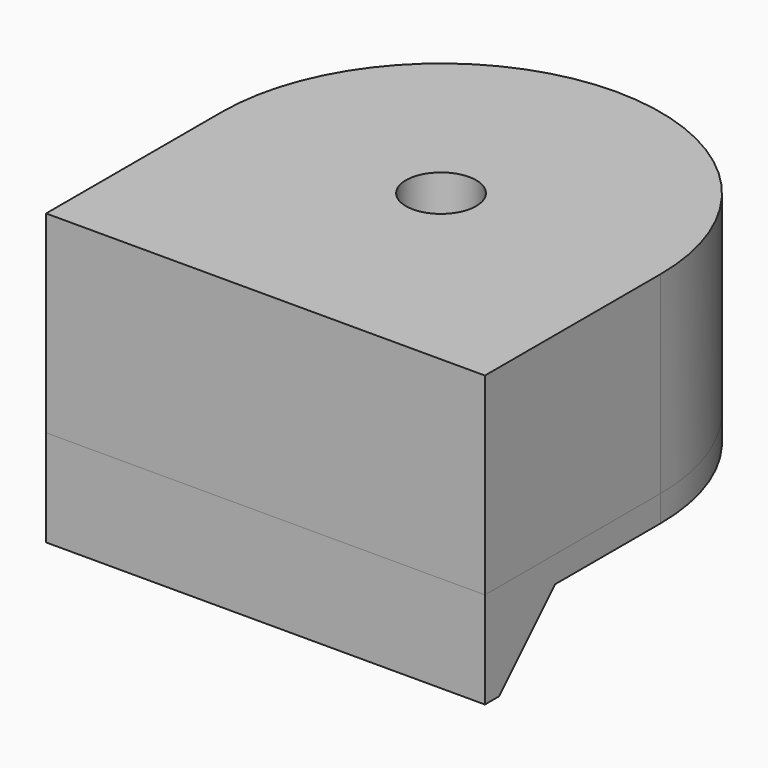
from build123d import *

# Parameters (mm, degrees)
F1_R     = 2
F2_DEPTH = 11
F3_DEPTH = 1.5
F5_DEPTH = 5.5
F6_SIZE  = 3.99999


# Not quite as in the source:
# - a fillet or chamfer is up to 0.001 mm smaller than in the source, because OpenCascade refuses the exact size


with BuildPart() as f2:
    # F1 (on Top) → F2 (new body)
    with BuildSketch(Plane.XY):
        with BuildLine():
            ThreePointArc((-4.8989794856, -11.5), (-10.4280209908, -6.8924870849), (-12.5, 0))
            Line((-12.5, 0), (-12.5, -11.5))
            Line((-12.5, -11.5), (-4.8989794856, -11.5))
        make_face()
        with BuildLine():
            ThreePointArc((4.8989794856, -11.5), (10.4280209908, -6.8924870849), (12.5, 0))
            ThreePointArc((12.5, 0), (8.8388347648, 8.8388347648), (0, 12.5))
            ThreePointArc((0, 12.5), (-8.8388347648, 8.8388347648), (-12.5, 0))
            ThreePointArc((-12.5, 0), (-10.4280209908, -6.8924870849), (-4.8989794856, -11.5))
            Line((-4.8989794856, -11.5), (4.8989794856, -11.5))
        make_face()
        Circle(F1_R, mode=Mode.SUBTRACT)
        with BuildLine():
            Line((12.5, -11.5), (12.5, 0))
            ThreePointArc((12.5, 0), (10.4280209908, -6.8924870849), (4.8989794856, -11.5))
            Line((4.8989794856, -11.5), (12.5, -11.5))
        make_face()
        with BuildLine():
            Line((-12.5, -12.5), (0, -12.5))
            ThreePointArc((0, -12.5), (-2.5, -12.2474487139), (-4.8989794856, -11.5))
            Line((-4.8989794856, -11.5), (-12.5, -11.5))
            Line((-12.5, -11.5), (-12.5, -12.5))
        make_face()
        with BuildLine():
            ThreePointArc((0, -12.5), (2.5, -12.2474487139), (4.8989794856, -11.5))
            Line((4.8989794856, -11.5), (-4.8989794856, -11.5))
            ThreePointArc((-4.8989794856, -11.5), (-2.5, -12.2474487139), (0, -12.5))
        make_face()
        with BuildLine():
            Line((12.5, -11.5), (4.8989794856, -11.5))
            ThreePointArc((4.8989794856, -11.5), (2.5, -12.2474487139), (0, -12.5))
            Line((0, -12.5), (12.5, -12.5))
            Line((12.5, -12.5), (12.5, -11.5))
        make_face()
    extrude(amount=F2_DEPTH)


with BuildPart() as f3:
    # F1 (on Top) → F3 (new body)
    with BuildSketch(Plane.XY):
        with BuildLine():
            Line((-12.5, -12.5), (0, -12.5))
            ThreePointArc((0, -12.5), (-2.5, -12.2474487139), (-4.8989794856, -11.5))
            Line((-4.8989794856, -11.5), (-12.5, -11.5))
            Line((-12.5, -11.5), (-12.5, -12.5))
        make_face()
        with BuildLine():
            ThreePointArc((0, -12.5), (2.5, -12.2474487139), (4.8989794856, -11.5))
            Line((4.8989794856, -11.5), (-4.8989794856, -11.5))
            ThreePointArc((-4.8989794856, -11.5), (-2.5, -12.2474487139), (0, -12.5))
        make_face()
        with BuildLine():
            Line((12.5, -11.5), (4.8989794856, -11.5))
            ThreePointArc((4.8989794856, -11.5), (2.5, -12.2474487139), (0, -12.5))
            Line((0, -12.5), (12.5, -12.5))
            Line((12.5, -12.5), (12.5, -11.5))
        make_face()
        with BuildLine():
            Line((12.5, -11.5), (12.5, 0))
            ThreePointArc((12.5, 0), (10.4280209908, -6.8924870849), (4.8989794856, -11.5))
            Line((4.8989794856, -11.5), (12.5, -11.5))
        make_face()
        with BuildLine():
            ThreePointArc((4.8989794856, -11.5), (10.4280209908, -6.8924870849), (12.5, 0))
            ThreePointArc((12.5, 0), (8.8388347648, 8.8388347648), (0, 12.5))
            ThreePointArc((0, 12.5), (-8.8388347648, 8.8388347648), (-12.5, 0))
            ThreePointArc((-12.5, 0), (-10.4280209908, -6.8924870849), (-4.8989794856, -11.5))
            Line((-4.8989794856, -11.5), (4.8989794856, -11.5))
        make_face()
        Circle(F1_R, mode=Mode.SUBTRACT)
        with BuildLine():
            ThreePointArc((-4.8989794856, -11.5), (-10.4280209908, -6.8924870849), (-12.5, 0))
            Line((-12.5, 0), (-12.5, -11.5))
            Line((-12.5, -11.5), (-4.8989794856, -11.5))
        make_face()
    extrude(amount=-F3_DEPTH)

    # F1 (on Top) → F5 (join)
    with BuildSketch(Plane.XY):
        with BuildLine():
            Line((-12.5, -12.5), (0, -12.5))
            ThreePointArc((0, -12.5), (-2.5, -12.2474487139), (-4.8989794856, -11.5))
            Line((-4.8989794856, -11.5), (-12.5, -11.5))
            Line((-12.5, -11.5), (-12.5, -12.5))
        make_face()
        with BuildLine():
            ThreePointArc((0, -12.5), (2.5, -12.2474487139), (4.8989794856, -11.5))
            Line((4.8989794856, -11.5), (-4.8989794856, -11.5))
            ThreePointArc((-4.8989794856, -11.5), (-2.5, -12.2474487139), (0, -12.5))
        make_face()
        with BuildLine():
            Line((12.5, -11.5), (4.8989794856, -11.5))
            ThreePointArc((4.8989794856, -11.5), (2.5, -12.2474487139), (0, -12.5))
            Line((0, -12.5), (12.5, -12.5))
            Line((12.5, -12.5), (12.5, -11.5))
        make_face()
    extrude(amount=-F5_DEPTH)

    # F6 (size 4 in the source; OpenCascade refuses exactly that, so slightly less here)
    f6_edges = [f3.edges().sort_by_distance(p)[0] for p in [
        (0, -11.5, -1.5),
    ]]
    chamfer(f6_edges, length=F6_SIZE)


solid = Compound([f2.part, f3.part])
